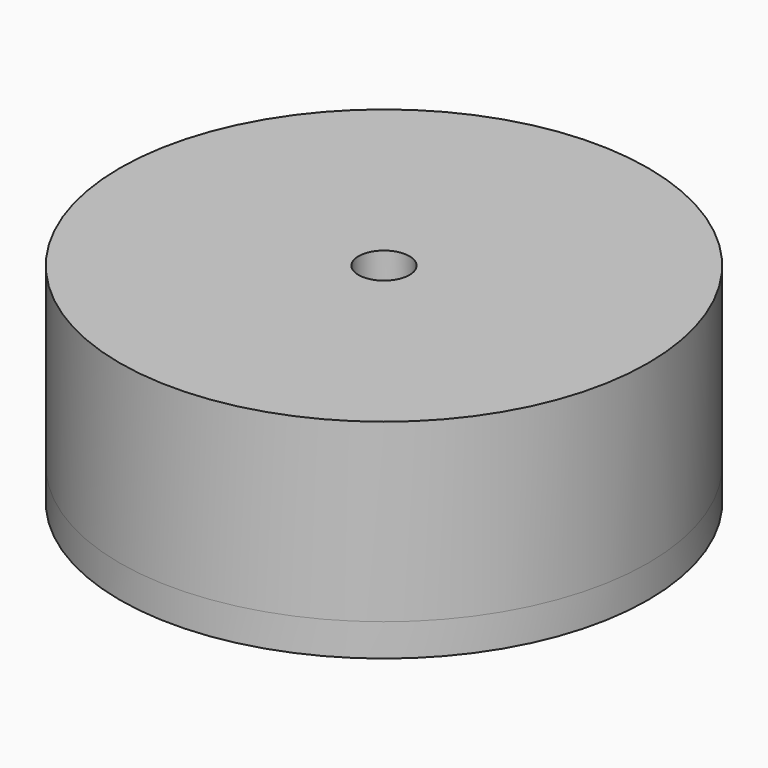
from build123d import *

# Parameters (mm, degrees)
F0_R     = 28.5
F1_DEPTH = 11
F3_DEPTH = 1
F4_R     = 2.75
F5_DEPTH = 6.4
F6_DEPTH = 8
F7_R     = 28.5
F7_R_2   = 27
F8_DEPTH = 4
F10_SIZE = 2


# Not quite as in the source:
# - a fillet or chamfer that OpenCascade refuses, or shapes differently, is made with other operations: its cross-section is extruded or revolved along the edge and cut away or added


with BuildPart() as f1:
    # F0 (on Top) → F1 (new body)
    with BuildSketch(Plane.XY):
        Circle(F0_R)
    extrude(amount=F1_DEPTH)

    # F2 (on face) → F3 (cut)
    with BuildSketch(Plane(origin=(0, 0, 0), x_dir=(1, 0, 0), z_dir=(0, 0, -1))):
        Polygon((10.68097998, 18.5), (-10.68097998, 18.5), (-21.36195996, 0), (-10.68097998, -18.5), (10.68097998, -18.5), (21.36195996, 0), align=None)
    extrude(amount=-F3_DEPTH, mode=Mode.SUBTRACT)

    # F4 (on face) → F5 (cut)
    with BuildSketch(Plane.XY.offset(11)):
        Circle(F4_R)
    extrude(amount=-F5_DEPTH, mode=Mode.SUBTRACT)

    # F6 (add): a face of the model
    f6_faces = [f1.faces().sort_by_distance(p)[0] for p in [
        (-27.6938982694, 0, 0),
    ]]
    extrude(f6_faces, amount=F6_DEPTH)

    # F7 (on face) → F8 (join)
    with BuildSketch(Plane(origin=(0, 0, -8), x_dir=(1, 0, 0), z_dir=(0, 0, -1))):
        Circle(F7_R)
        Circle(F7_R_2, mode=Mode.SUBTRACT)
    extrude(amount=F8_DEPTH)

    # F9: chamfer of 2 on 1 edges, made by hand

    # F9_s1 → F9_t2 (revolve, cut)
    with BuildSketch(Plane.XZ):
        Polygon((29, -12), (27, -10), (27, -12), align=None)
    revolve(axis=Axis((0, 0, -12), (0, 0, -1)), mode=Mode.SUBTRACT)

    # F10
    f10_edges = [f1.edges().sort_by_distance(p)[0] for p in [
        (0, -18.5, -8),
        (16.02147, -9.25, -8),
        (16.02147, 9.25, -8),
        (0, 18.5, -8),
        (-16.02147, 9.25, -8),
        (-16.02147, -9.25, -8),
    ]]
    chamfer(f10_edges, length=F10_SIZE)


solid = f1.part
